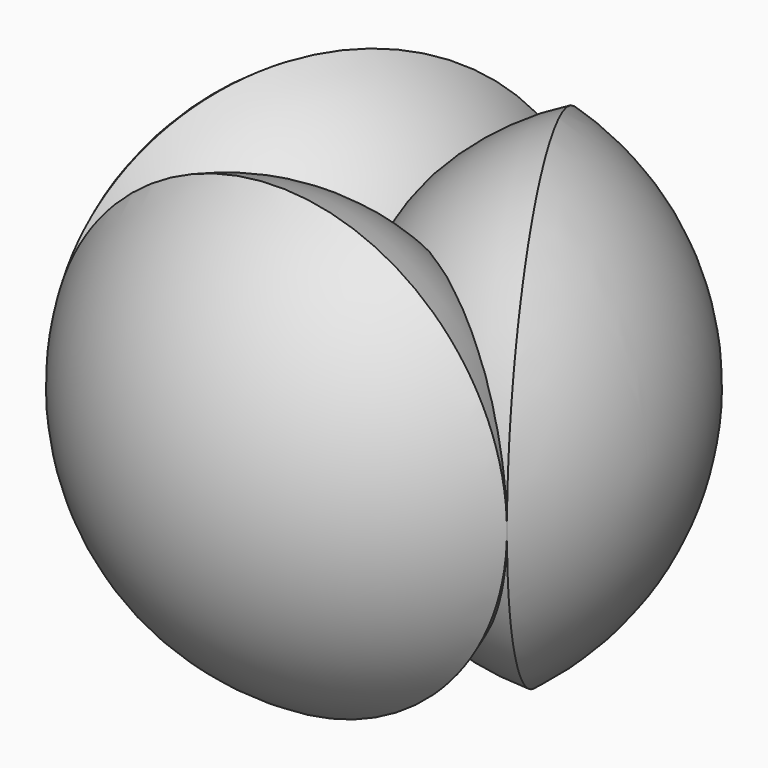
from build123d import *

# Parameters (mm, degrees)
F6_COUNT = 3


# Not quite as in the source:
# - a feature of the source that left no trace in its solid (it failed there, or was rolled back) is left out


with BuildPart() as f5:
    # F4 (on Top) → F5 (revolve)
    with BuildSketch(Plane.XY):
        with BuildLine():
            Line((-16.6504235141, -9.613126498), (181.628262935, 104.863126498))
            ThreePointArc((181.628262935, 104.863126498), (25.2507932125, 146.7643432246), (-16.6504235141, -9.613126498))
        make_face()
    revolve(axis=Axis((82.4889197105, 47.625, 0), (0.8660254038, 0.5, 0)))


with BuildPart() as f6_1:
    # F6: instance of F5
    add(f5.part.rotate(Axis((0, 0, 36.1574739218), (0, 0, 1)), 1 * 360 / F6_COUNT))


with BuildPart() as f6_2:
    # F6: instance of F5
    add(f5.part.rotate(Axis((0, 0, 36.1574739218), (0, 0, 1)), 2 * 360 / F6_COUNT))


with BuildPart() as f10_tool:
    # F9 (on Front) → F10 (revolve)
    with BuildSketch(Plane.XZ):
        with BuildLine():
            Line((-127, 0), (127, 0))
            ThreePointArc((127, 0), (0, 127), (-127, 0))
        make_face()
    revolve(axis=Axis((0, 0, 0), (1, 0, 0)))


with BuildPart() as f5_1:
    add(f5.part)

    # F10: intersect by f10_tool
    add(f10_tool.part, mode=Mode.INTERSECT)


with BuildPart() as f6_1_1:
    add(f6_1.part)

    # F10: intersect by f10_tool
    add(f10_tool.part, mode=Mode.INTERSECT)


with BuildPart() as f6_2_1:
    add(f6_2.part)

    # F10: intersect by f10_tool
    add(f10_tool.part, mode=Mode.INTERSECT)


solid = Compound([f5_1.part, f6_1_1.part, f6_2_1.part])
